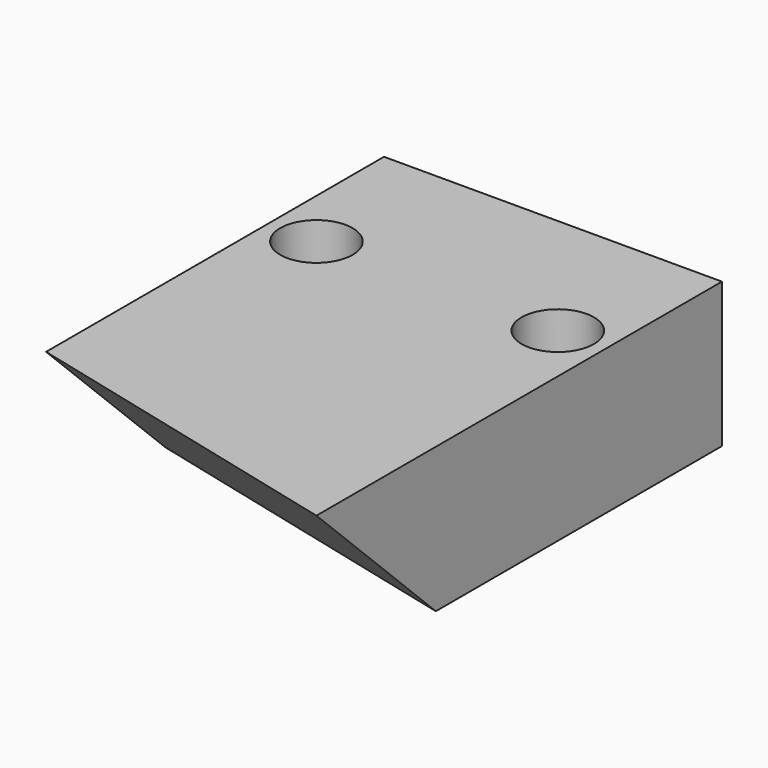
from build123d import *

# Parameters (mm, degrees)
F1_DEPTH = 6
F2_SIZE  = 5.99999
F3_R     = 1.5
F4_DEPTH = 6


# Not quite as in the source:
# - a fillet or chamfer is up to 0.001 mm smaller than in the source, because OpenCascade refuses the exact size


with BuildPart() as f1:
    # F0 (on Top) → F1 (new body)
    with BuildSketch(Plane.XY):
        Polygon((10.2662842423, 7.4127185345), (-3.7337157577, 7.4127185345), (-3.7337157577, -10.0872814655), (10.2662842423, -13.5872814655), align=None)
    extrude(amount=F1_DEPTH)

    # F2 (size 6 in the source; OpenCascade refuses exactly that, so slightly less here)
    f2_edges = [f1.edges().sort_by_distance(p)[0] for p in [
        (3.266284, -11.837281, 0),
    ]]
    chamfer(f2_edges, length=F2_SIZE)

    # F3 (on face) → F4 (cut, through all)
    with BuildSketch(Plane.XY.offset(6)):
        with Locations((-1.7337157577, 1.4127185345)):
            Circle(F3_R)
        with Locations((8.2662842423, 1.4127185345)):
            Circle(F3_R)
    extrude(amount=-F4_DEPTH, mode=Mode.SUBTRACT)


solid = f1.part
